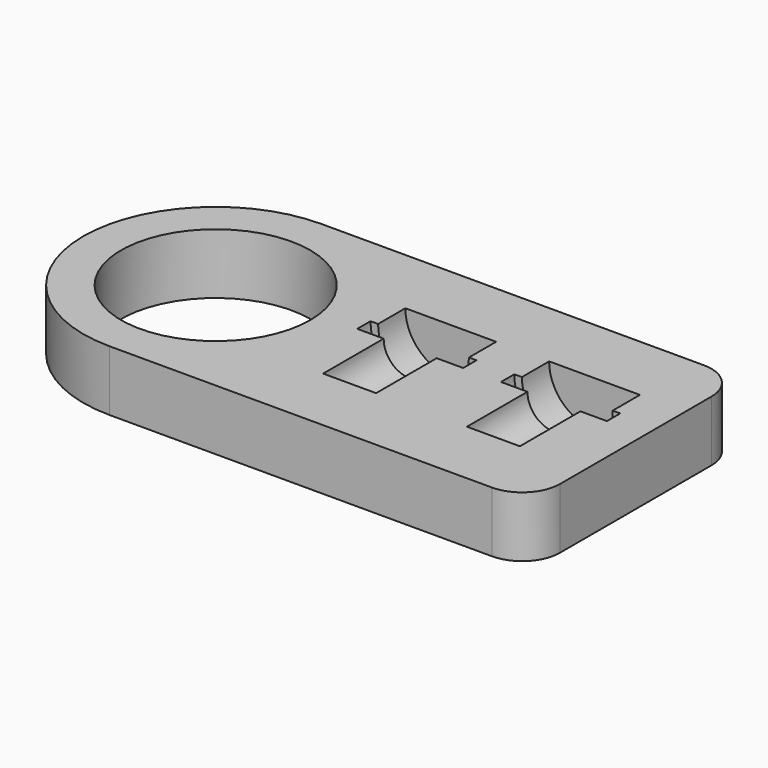
from build123d import *

# Parameters (mm, degrees)
F0_R         = 12.5
F1_DEPTH     = 8
F5_TEXT_SIZE = 5.5555555556
F6_DEPTH     = 1


# Not quite as in the source:
# - Text() gives the source's letters only with a copy of the font that has no kerning and outlines rounded to 1/6400 em; it was checked with that copy


with BuildPart() as f1:
    # F0 (on Top) → F1 (new body)
    with BuildSketch(Plane.XY):
        with BuildLine():
            ThreePointArc((0, 17.5), (5.1256313292, 5.1256313292), (17.5, 0))
            Line((17.5, 0), (68, 0))
            ThreePointArc((68, 0), (71.5355339059, 1.4644660941), (73, 5))
            Line((73, 5), (73, 30))
            ThreePointArc((73, 30), (71.5355339059, 33.5355339059), (68, 35))
            Line((68, 35), (17.5, 35))
            ThreePointArc((17.5, 35), (5.1256313292, 29.8743686708), (0, 17.5))
        make_face()
        with Locations((17.5, 17.5)):
            Circle(F0_R, mode=Mode.SUBTRACT)
    extrude(amount=F1_DEPTH)

    # F2 (on face) → F3 (revolve, cut)
    with BuildSketch(Plane.XY.offset(8)):
        Polygon((42, 19), (42, 9), (45.5, 9), (45.5, 19), (49, 19), (49, 21.2), (48, 21.2), (48, 25.7), (42, 25.7), (42, 21.2), align=None)
    revolve(axis=Axis((42, 14, 8), (0, 1, 0)), mode=Mode.SUBTRACT)

    # F2 (on face) → F4 (revolve, cut)
    with BuildSketch(Plane.XY.offset(8)):
        Polygon((61, 19), (61, 9), (64.5, 9), (64.5, 19), (68, 19), (68, 21.2), (67, 21.2), (67, 25.7), (61, 25.7), (61, 21.2), align=None)
    revolve(axis=Axis((61, 14, 8), (0, 1, 0)), mode=Mode.SUBTRACT)

    # F5 (on face) → F6 (cut)
    with BuildSketch(Plane(origin=(0, 0, 0), x_dir=(1, 0, 0), z_dir=(0, 0, -1))):
        with Locations((30, -9)):
            Text('1051', F5_TEXT_SIZE, font='Open Sans', text_align=(TextAlign.LEFT, TextAlign.BOTTOM))
    extrude(amount=-F6_DEPTH, mode=Mode.SUBTRACT)


solid = f1.part
